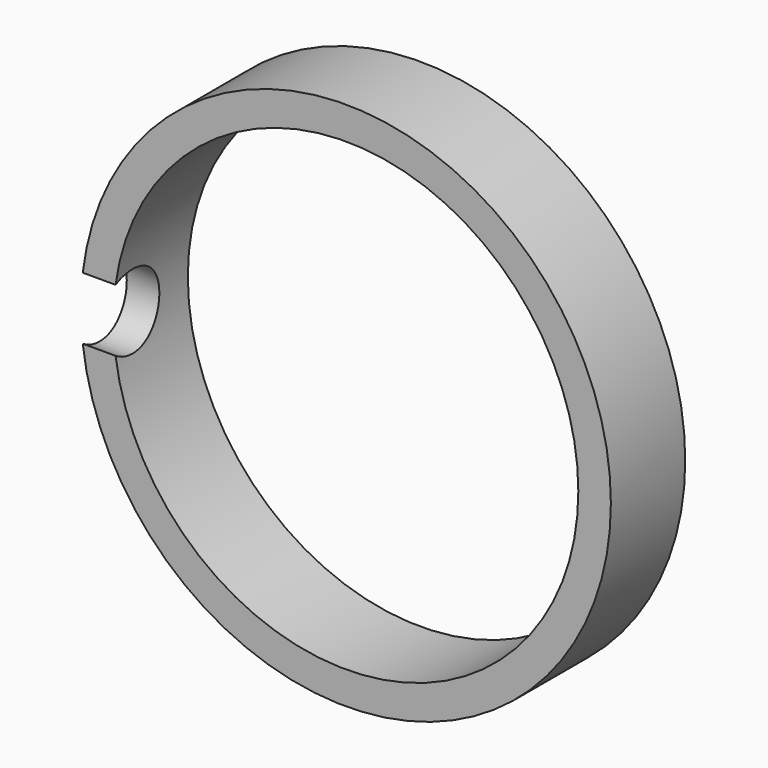
from build123d import *

# Parameters (mm, degrees)
F0_R     = 28.5
F0_R_2   = 25
F1_DEPTH = 10
F3_D     = 8
F3_DEPTH = 28.501


with BuildPart() as f1:
    # F0 (on Front) → F1 (new body)
    with BuildSketch(Plane.XZ):
        Circle(F0_R)
        Circle(F0_R_2, mode=Mode.SUBTRACT)
    extrude(amount=F1_DEPTH)

    # F3 (through all, one way)
    with BuildSketch(Plane.YZ):
        with Locations((-7.8321313486, 0)):
            Circle(F3_D / 2)
    extrude(amount=-F3_DEPTH, mode=Mode.SUBTRACT)


solid = f1.part
